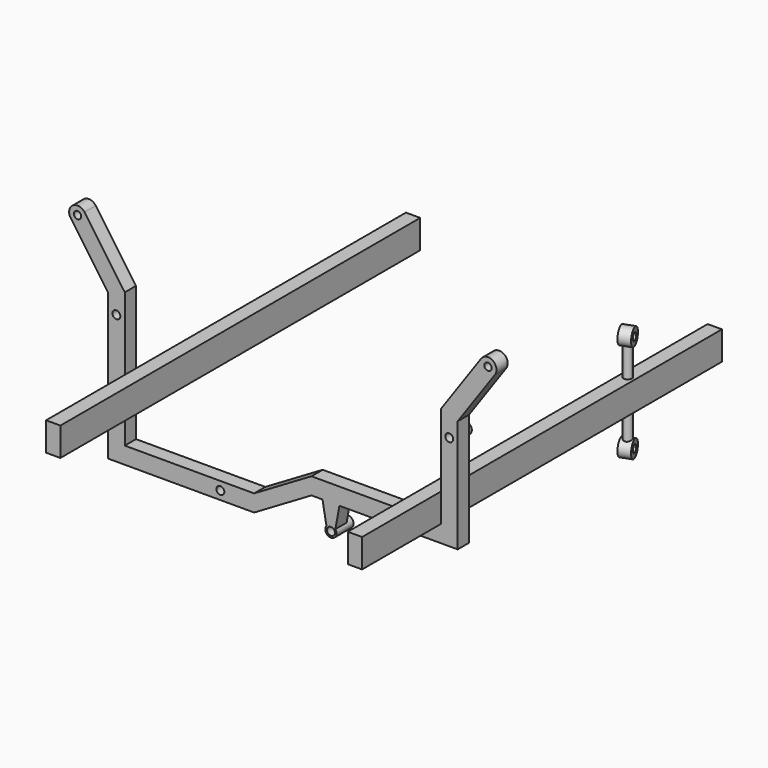
from build123d import *

# Parameters (mm, degrees)
F0_R          = 7
F0_R_2        = 6.5
F1_DEPTH      = 25
F2_W          = 25.4
F2_H          = 50.8
F3_DEPTH      = 200
F3_DEPTH_BACK = 600
F6_DEPTH      = 65
F8_R          = 15
F8_R_2        = 7
F9_DEPTH      = 10
F10_R         = 15
F10_R_2       = 7
F11_DEPTH     = 10
F12_R         = 7.5
F13_REACH     = 111.2142034356
F14_R         = 10
F14_R_2       = 7
F15_DEPTH     = 12.7
F16_R         = 10
F16_R_2       = 7
F17_DEPTH     = 12.7


with BuildPart() as f1:
    # F0 (on Front) → F1 (new body)
    with BuildSketch(Plane.XZ):
        with BuildLine():
            Line((-230, 0), (-301.7204504189, 102.2319018363))
            ThreePointArc((-301.7204504189, 102.2319018363), (-322.6146771319, 105.8967742855), (-326.2795495811, 85.0025475726))
            Line((-326.2795495811, 85.0025475726), (-260, -9.4737749679))
            Line((-260, -9.4737749679), (-260, -270))
            Line((-260, -270), (0, -270))
            Line((0, -270), (102, -210))
            Line((102, -210), (121.6, -210))
            Line((121.6, -210), (128.6, -249))
            ThreePointArc((128.6, -249), (136.6, -265), (144.6, -249))
            Line((144.6, -249), (151.6, -210))
            Line((151.6, -210), (362, -210))
            Line((362, -210), (362, -9.4737749679))
            Line((362, -9.4737749679), (428.2795495811, 85.0025475726))
            ThreePointArc((428.2795495811, 85.0025475726), (424.6146771319, 105.8967742855), (403.7204504189, 102.2319018363))
            Line((403.7204504189, 102.2319018363), (332, 0))
            Line((332, 0), (332, -129.2))
            Line((332, -129.2), (332, -180))
            Line((332, -180), (306.6, -180))
            Line((306.6, -180), (102, -180))
            Line((102, -180), (0, -240))
            Line((0, -240), (-230, -240))
            Line((-230, -240), (-230, 0))
        make_face()
        with Locations((-60, -255)):
            Circle(F0_R, mode=Mode.SUBTRACT)
        with Locations((136.6, -255)):
            Circle(F0_R, mode=Mode.SUBTRACT)
        with Locations((-245, -40)):
            Circle(F0_R, mode=Mode.SUBTRACT)
        with Locations((-314, 93.6172247045)):
            Circle(F0_R_2, mode=Mode.SUBTRACT)
        with Locations((347, -40)):
            Circle(F0_R, mode=Mode.SUBTRACT)
        with Locations((416, 93.6172247045)):
            Circle(F0_R_2, mode=Mode.SUBTRACT)
    extrude(amount=F1_DEPTH)

    # F2 (on Front) → F3 (join, two sides)
    with BuildSketch(Plane.XZ) as f3_sk:
        with Locations((319.3, -154.6)):
            Rectangle(F2_W, F2_H)
        with Locations((-217.3, -154.6)):
            Rectangle(F2_W, F2_H)
    extrude(amount=F3_DEPTH)
    extrude(f3_sk.sketch, amount=-F3_DEPTH_BACK)

    # F5 (on face) → F6 (join)
    with BuildSketch(Plane.XY.offset(-129.2)):
        with BuildLine():
            ThreePointArc((316.7348489251, 413.4476946559), (314.9981767274, 400.2563596678), (326.8, 406.4))
            ThreePointArc((326.8, 406.4), (323.6018232726, 412.5436403322), (316.7348489251, 413.4476946559))
        make_face()
    extrude(amount=F6_DEPTH)

    # F8 (on face) → F9 (join, symmetric)
    with BuildSketch(Plane(origin=(412.5634376322, 150.1608110447, 0), x_dir=(0.3420201433, -0.9396926208, 0), z_dir=(-0.9396926208, -0.3420201433, 0))):
        with Locations((-272.6840493235, -64.6)):
            Circle(F8_R)
        with Locations((-272.6840493235, -64.6)):
            Circle(F8_R_2, mode=Mode.SUBTRACT)
    extrude(amount=F9_DEPTH, both=True)



with BuildPart() as f11:
    # F10 (on face) → F11 (new body, symmetric)
    with BuildSketch(Plane(origin=(412.5634376322, 150.1608110447, 0), x_dir=(0.3420201433, -0.9396926208, 0), z_dir=(-0.9396926208, -0.3420201433, 0))):
        with Locations((-272.6840493235, -240)):
            Circle(F10_R)
        with Locations((-272.6840493235, -240)):
            Circle(F10_R_2, mode=Mode.SUBTRACT)
    extrude(amount=F11_DEPTH, both=True)


with BuildPart() as f1_1:
    add(f1.part)

    add(f11.part)  # F13 merges F11
    f13_end = f1_1.faces().sort_by_distance((314.1696978501, 420.4953893118, -240))[0]
    # F12 (on face) → F13 (join, up to a face of the model that its end follows)
    with BuildSketch(Plane(origin=(0, 0, -180), x_dir=(1, 0, 0), z_dir=(0, 0, -1))):
        with Locations((319.3, -406.4)):
            Circle(F12_R)
    f13_long = extrude(amount=F13_REACH, mode=Mode.PRIVATE)
    add(split(f13_long, bisect_by=f13_end, keep=Keep.ALL, mode=Mode.PRIVATE).solids().sort_by_distance((319.3, 406.4, -180))[0])

    # F14 (on face) → F15 (join)
    with BuildSketch(Plane.XZ):
        with Locations((136.6, -255)):
            Circle(F14_R)
        with Locations((136.6, -255)):
            Circle(F14_R_2, mode=Mode.SUBTRACT)
    extrude(amount=-F15_DEPTH)

    # F16 (on face) → F17 (join)
    with BuildSketch(Plane.XZ):
        with Locations((347, -40)):
            Circle(F16_R)
        with Locations((347, -40)):
            Circle(F16_R_2, mode=Mode.SUBTRACT)
    extrude(amount=-F17_DEPTH)


solid = f1_1.part
